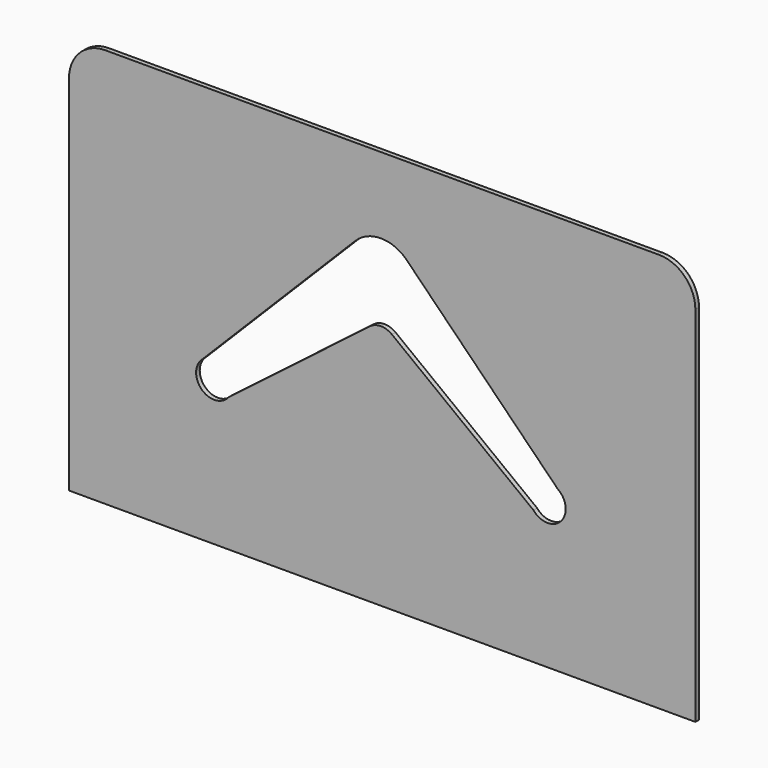
from build123d import *

# Parameters (mm, degrees)
F1_DEPTH = 1.5875


# Not quite as in the source:
# - ends of sketch curves that miss each other by under 0.0002 mm in the source are joined


with BuildPart() as f1:
    # F0 (on Front) → F1 (new body)
    with BuildSketch(Plane.XZ):
        with BuildLine():
            Line((97.284460747, 47.1963935311), (-96.390539253, 47.1963935311))
            ThreePointArc((-96.390539253, 47.1963935311), (-105.370795374, 43.4766496521), (-109.090539253, 34.4963935311))
            Line((-109.090539253, 34.4963935311), (-109.090539253, -92.5036064689))
            Line((-109.090539253, -92.5036064689), (109.984460747, -92.5036064689))
            Line((109.984460747, -92.5036064689), (109.984460747, 34.4963935311))
            ThreePointArc((109.984460747, 34.4963935311), (106.2647168681, 43.4766496521), (97.284460747, 47.1963935311))
        make_face()
        with BuildLine():
            ThreePointArc((-53.3636475136, -45.7096316546), (-62.7650367506, -46.2093108693), (-62.3307099384, -36.8046758885))
            Line((-62.3307099384, -36.8046758885), (-9.0114088008, 16.8864949952))
            ThreePointArc((-9.0114088008, 16.8864949952), (4.2539e-06, 20.6375), (9.0114147958, 16.8864889585))
            Line((9.0114147958, 16.8864889585), (61.8517940181, -36.4462340741))
            ThreePointArc((61.8517940181, -36.4462340741), (63.9001946683, -38.7279945788), (64.640539253, -41.7036064689))
            ThreePointArc((64.640539253, -41.7036064689), (60.4161847378, -47.6872618127), (53.3636475136, -45.7096316546))
            Line((53.3636475136, -45.7096316546), (3.8656210952, -7.7286783496))
            ThreePointArc((3.8656210952, -7.7286783496), (0, -6.4164827869), (-3.8656210952, -7.7286783496))
            Line((-3.8656210952, -7.7286783496), (-53.3636475136, -45.7096316546))
        make_face(mode=Mode.SUBTRACT)
    extrude(amount=F1_DEPTH)


solid = f1.part
